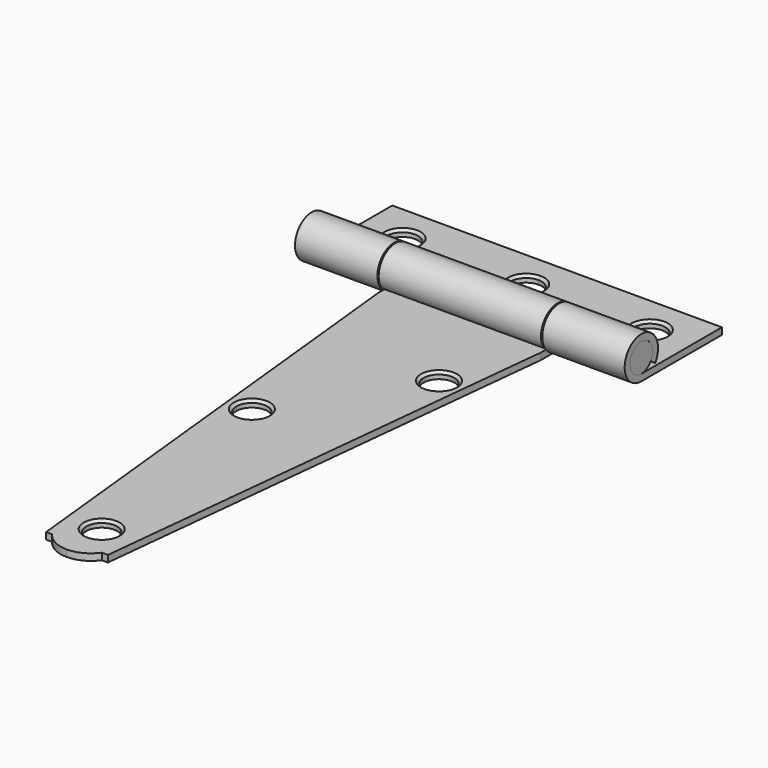
from build123d import *
from build123d import SkipClean  # not in build123d's __all__

# Parameters (mm, degrees)
F0_R          = 3
F1_DEPTH      = 1.3
F2_DEPTH      = 1.3
F5_DEPTH      = 1.301
F7_DEPTH      = 15.75
F7_DEPTH_BACK = 15.75
F9_DEPTH      = 16
F11_R         = 2.75
F12_DEPTH     = 64
F13_SIZE      = 0.5
F13_2_SIZE    = 0.5


with BuildPart() as f1:
    # F0 (on Top) → F1 (new body)
    with BuildSketch(Plane.XY):
        with BuildLine():
            Line((0, 15.5), (-32, 15.5))
            Line((-32, 15.5), (-32, 0))
            Line((-32, 0), (-16, 0))
            Line((-16, 0), (-16, 0.5))
            Line((-16, 0.5), (0, 0.5))
            Line((0, 0.5), (0, 5))
            ThreePointArc((0, 5), (-3, 8), (0, 11))
            Line((0, 11), (0, 15.5))
        make_face()
        with Locations((-24, 8)):
            Circle(F0_R, mode=Mode.SUBTRACT)
    extrude(amount=F1_DEPTH)

    # F3: F1 across face


with BuildPart() as f2:
    # F0 (on Top) → F2 (new body)
    with BuildSketch(Plane.XY):
        with BuildLine():
            Line((0, -92), (0, -8.1))
            Line((0, -8.1), (-15.75, -8.1))
            Line((-15.75, -8.1), (-6, -101))
            Line((-6, -101), (-4.8112012446, -101))
            ThreePointArc((-4.8112012446, -101), (-2.7109803308, -102.8376972935), (0, -103.5))
            Line((0, -103.5), (0, -98))
            ThreePointArc((0, -98), (-3, -95), (0, -92))
        make_face()
        with Locations((-6.8525296017, -50)):
            Circle(F0_R, mode=Mode.SUBTRACT)
        with Locations((-6.8525296017, -50)):
            Circle(F0_R)
    extrude(amount=F2_DEPTH)

    # F4: F2 across face


with BuildPart() as f1_1:
    add(f1.part, clean=False)
    with SkipClean():  # cleaning this boolean's faces spoils the solid; the shape is the same uncleaned
        add(f1.part.mirror(Plane(origin=(0, -50.05, 0.65), x_dir=(0, 1, 0), z_dir=(1, 0, 0))), clean=False)

    # F8 (on face) → F9 (join, through all)
    with BuildSketch(Plane(origin=(-32, 0, 0), x_dir=(0, -1, 0), z_dir=(-1, 0, 0))):
        with BuildLine():
            Line((0, 0), (4.05, 0))
            ThreePointArc((4.05, 0), (5.9458344619, 7.6288701699), (0.6994096777, 1.7749078058))
            Line((0.6994096777, 1.7749078058), (1.7749078058, 2.5051843126))
            ThreePointArc((1.7749078058, 2.5051843126), (5.337295005, 6.480097029), (4.05, 1.3))
            Line((4.05, 1.3), (0, 1.3))
            Line((0, 1.3), (0, 0))
        make_face()
    extrude(amount=-F9_DEPTH)

    # F10: F1 across plane


with BuildPart() as f2_1:
    add(f2.part, clean=False)
    with SkipClean():  # cleaning this boolean's faces spoils the solid; the shape is the same uncleaned
        add(f2.part.mirror(Plane(origin=(0, -50.05, 0.65), x_dir=(0, 1, 0), z_dir=(1, 0, 0))), clean=False)

    # F0 (on Top) → F5 (cut, through all)
    with BuildSketch(Plane.XY):
        with Locations((9.4763186222, -25)):
            Circle(F0_R)
        with Locations((-6.8525296017, -50)):
            Circle(F0_R)
    extrude(amount=F5_DEPTH, mode=Mode.SUBTRACT)

    # F6 (on Right) → F7 (join, two sides)
    with BuildSketch(Plane.YZ) as f7_sk:
        with BuildLine():
            Line((-8.1, 0), (-4.05, 0))
            ThreePointArc((-4.05, 0), (-2.1541655381, 7.6288701699), (-7.4005903223, 1.7749078058))
            Line((-7.4005903223, 1.7749078058), (-6.3250921942, 2.5051843126))
            ThreePointArc((-6.3250921942, 2.5051843126), (-2.762704995, 6.480097029), (-4.05, 1.3))
            Line((-4.05, 1.3), (-8.1, 1.3))
            Line((-8.1, 1.3), (-8.1, 0))
        make_face()
    extrude(amount=F7_DEPTH)
    extrude(f7_sk.sketch, amount=-F7_DEPTH_BACK)

    # F13#2
    f13_2_edges = [f2_1.edges().sort_by_distance(p)[0] for p in [
        (6.476319, -25, 1.3),
        (-9.85253, -50, 1.3),
        (-3, -95, 1.3),
        (3, -95, 1.3),
    ]]
    chamfer(f13_2_edges, length=F13_2_SIZE)


with BuildPart() as f1_2:
    add(f1_1.part, clean=False)
    add(f1_1.part.mirror(Plane.YZ), clean=False)

    # F13
    f13_edges = [f1_2.edges().sort_by_distance(p)[0] for p in [
        (27, 8, 1.3),
        (-3, 8, 1.3),
        (3, 8, 1.3),
        (-27, 8, 1.3),
    ]]
    chamfer(f13_edges, length=F13_SIZE)


with BuildPart() as f12:
    # F11 (on face) → F12 (new body, through all)
    with BuildSketch(Plane(origin=(-32, 0, 0), x_dir=(0, -1, 0), z_dir=(-1, 0, 0))):
        with Locations((4.05, 4.05)):
            Circle(F11_R)
    extrude(amount=-F12_DEPTH)


solid = Compound([f2_1.part, f1_2.part, f12.part])
